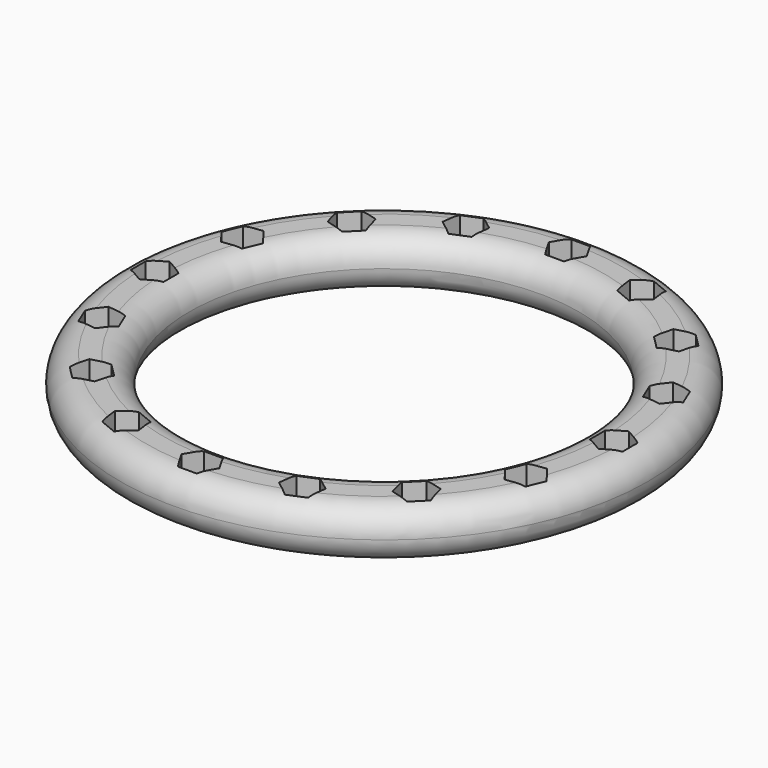
from build123d import *

# Parameters (mm, degrees)
F0_W     = 15
F0_H     = 11
F3_DEPTH = 8.5


# Not quite as in the source:
# - a fillet or chamfer that OpenCascade refuses, or shapes differently, is made with other operations: its cross-section is extruded or revolved along the edge and cut away or added


with BuildPart() as f1:
    # F0 (on Front) → F1 (revolve)
    with BuildSketch(Plane.XZ):
        with Locations((50, 5.5)):
            Rectangle(F0_W, F0_H)
    revolve(axis=Axis((0, 0, 11.3872010261), (0, 0, 1)))

    # F2 (on face) → F3 (cut)
    with BuildSketch(Plane.XY.offset(11)):
        Polygon((-2.0640272124, 46.425), (2.0640272124, 46.425), (4.1280544247, 50), (2.0640272124, 53.575), (-2.0640272124, 53.575), (-4.1280544247, 50), align=None)
        Polygon((-15.8591658515, 43.680976315), (-15.3203466262, 47.7737146618), (-18.5953523929, 50.2867149724), (-22.409177385, 48.7069769362), (-22.9479966103, 44.6142385893), (-19.6729908436, 42.1012382787), align=None)
        Polygon((-31.3679446782, 34.286919955), (-32.4363637825, 38.2743143361), (-36.4237581637, 39.3427334405), (-39.3427334405, 36.4237581637), (-38.2743143361, 32.4363637825), (-34.286919955, 31.3679446782), align=None)
        Polygon((-42.1012382787, 19.6729908436), (-44.6142385893, 22.9479966103), (-48.7069769362, 22.409177385), (-50.2867149724, 18.5953523929), (-47.7737146618, 15.3203466262), (-43.680976315, 15.8591658515), align=None)
        Polygon((-46.425, 2.0640272124), (-50, 4.1280544247), (-53.575, 2.0640272124), (-53.575, -2.0640272124), (-50, -4.1280544247), (-46.425, -2.0640272124), align=None)
        Polygon((-43.680976315, -15.8591658515), (-47.7737146618, -15.3203466262), (-50.2867149724, -18.5953523929), (-48.7069769362, -22.409177385), (-44.6142385893, -22.9479966103), (-42.1012382787, -19.6729908436), align=None)
        Polygon((-34.286919955, -31.3679446782), (-38.2743143361, -32.4363637825), (-39.3427334405, -36.4237581637), (-36.4237581637, -39.3427334405), (-32.4363637825, -38.2743143361), (-31.3679446782, -34.286919955), align=None)
        Polygon((-19.6729908436, -42.1012382787), (-22.9479966103, -44.6142385893), (-22.409177385, -48.7069769362), (-18.5953523929, -50.2867149724), (-15.3203466262, -47.7737146618), (-15.8591658515, -43.680976315), align=None)
        Polygon((-2.0640272124, -46.425), (-4.1280544247, -50), (-2.0640272124, -53.575), (2.0640272124, -53.575), (4.1280544247, -50), (2.0640272124, -46.425), align=None)
        Polygon((15.8591658515, -43.680976315), (15.3203466262, -47.7737146618), (18.5953523929, -50.2867149724), (22.409177385, -48.7069769362), (22.9479966103, -44.6142385893), (19.6729908436, -42.1012382787), align=None)
        Polygon((31.3679446782, -34.286919955), (32.4363637825, -38.2743143361), (36.4237581637, -39.3427334405), (39.3427334405, -36.4237581637), (38.2743143361, -32.4363637825), (34.286919955, -31.3679446782), align=None)
        Polygon((42.1012382787, -19.6729908436), (44.6142385893, -22.9479966103), (48.7069769362, -22.409177385), (50.2867149724, -18.5953523929), (47.7737146618, -15.3203466262), (43.680976315, -15.8591658515), align=None)
        Polygon((46.425, -2.0640272124), (50, -4.1280544247), (53.575, -2.0640272124), (53.575, 2.0640272124), (50, 4.1280544247), (46.425, 2.0640272124), align=None)
        Polygon((43.680976315, 15.8591658515), (47.7737146618, 15.3203466262), (50.2867149724, 18.5953523929), (48.7069769362, 22.409177385), (44.6142385893, 22.9479966103), (42.1012382787, 19.6729908436), align=None)
        Polygon((34.286919955, 31.3679446782), (38.2743143361, 32.4363637825), (39.3427334405, 36.4237581637), (36.4237581637, 39.3427334405), (32.4363637825, 38.2743143361), (31.3679446782, 34.286919955), align=None)
        Polygon((19.6729908436, 42.1012382787), (22.9479966103, 44.6142385893), (22.409177385, 48.7069769362), (18.5953523929, 50.2867149724), (15.3203466262, 47.7737146618), (15.8591658515, 43.680976315), align=None)
    extrude(amount=-F3_DEPTH, mode=Mode.SUBTRACT)

    # F4: fillet of radius 5.5 on 4 edges, made by hand

    # F4_s1 → F4_t2 (revolve, cut)
    with BuildSketch(Plane.XZ):
        with BuildLine():
            ThreePointArc((48, 11), (44.1109127035, 9.3890872965), (42.5, 5.5))
            Line((42.5, 5.5), (42.5, 11))
            Line((42.5, 11), (48, 11))
        make_face()
    revolve(axis=Axis((0, 0, 11), (0, 0, 1)), mode=Mode.SUBTRACT)

    # F4_s3 → F4_t4 (revolve, cut)
    with BuildSketch(Plane.XZ):
        with BuildLine():
            ThreePointArc((52, 11), (55.8890872965, 9.3890872965), (57.5, 5.5))
            Line((57.5, 5.5), (57.5, 11))
            Line((57.5, 11), (52, 11))
        make_face()
    revolve(axis=Axis((0, 0, 11), (0, 0, 1)), mode=Mode.SUBTRACT)

    # F4_s5 → F4_t6 (revolve, cut)
    with BuildSketch(Plane.XZ):
        with BuildLine():
            ThreePointArc((57.5, 5.5), (55.8890872965, 1.6109127035), (52, 0))
            Line((52, 0), (57.5, 0))
            Line((57.5, 0), (57.5, 5.5))
        make_face()
    revolve(axis=Axis((0, 0, 0), (0, 0, 1)), mode=Mode.SUBTRACT)

    # F4_s7 → F4_t8 (revolve, cut)
    with BuildSketch(Plane.XZ):
        with BuildLine():
            ThreePointArc((42.5, 5.5), (44.1109127035, 1.6109127035), (48, 0))
            Line((48, 0), (42.5, 0))
            Line((42.5, 0), (42.5, 5.5))
        make_face()
    revolve(axis=Axis((0, 0, 0), (0, 0, 1)), mode=Mode.SUBTRACT)


solid = f1.part
